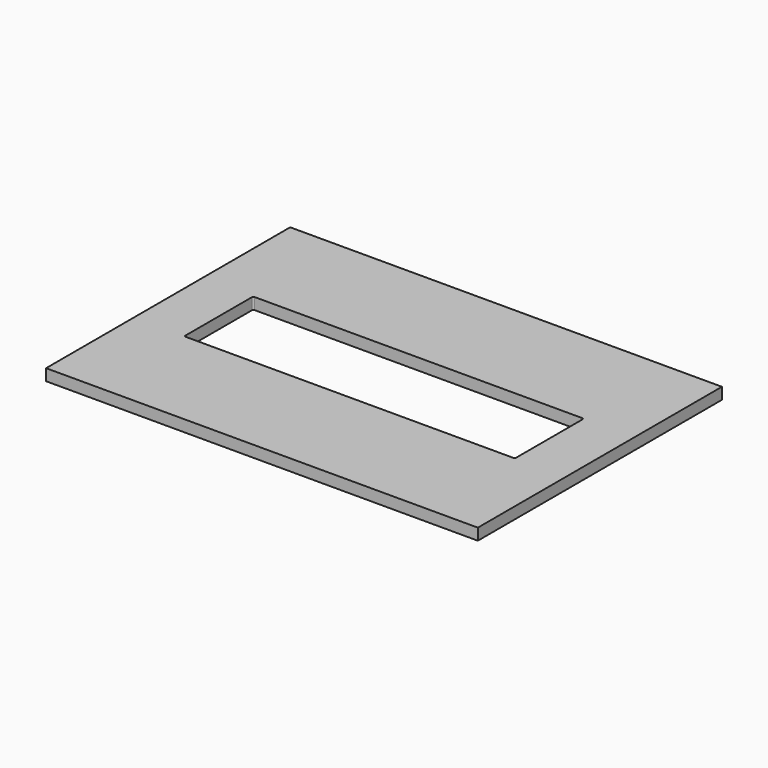
from build123d import *

# Parameters (mm, degrees)
F0_W     = 238.125
F0_H     = 168.275
F1_DEPTH = 6.35
F2_W     = 179.832
F2_H     = 44.958
F3_DEPTH = 25.4
F5_DEPTH = 6.351


# Not quite as in the source:
# - a feature of the source that left no trace in its solid (it failed there, or was rolled back) is left out


with BuildPart() as f1:
    # F0 (on Top) → F1 (new body)
    with BuildSketch(Plane.XY):
        Rectangle(F0_W, F0_H)
    extrude(amount=F1_DEPTH)

    # F2 (on face) → F3 (cut)
    with BuildSketch(Plane.XY.offset(6.35)):
        Rectangle(F2_W, F2_H)
    extrude(amount=-F3_DEPTH, mode=Mode.SUBTRACT)

    # F4 (on face) → F5 (cut, through all)
    with BuildSketch(Plane.XY.offset(6.35)):
        with BuildLine():
            Line((90.3986, 23.749), (-90.3986, 23.749))
            ThreePointArc((-90.3986, 23.749), (-90.9553758795, 23.5183758795), (-91.186, 22.9616))
            Line((-91.186, 22.9616), (-91.186, -22.9616))
            ThreePointArc((-91.186, -22.9616), (-90.9553758795, -23.5183758795), (-90.3986, -23.749))
            Line((-90.3986, -23.749), (90.3986, -23.749))
            ThreePointArc((90.3986, -23.749), (90.9553758795, -23.5183758795), (91.186, -22.9616))
            Line((91.186, -22.9616), (91.186, 22.9616))
            ThreePointArc((91.186, 22.9616), (90.9553758795, 23.5183758795), (90.3986, 23.749))
        make_face()
    extrude(amount=-F5_DEPTH, mode=Mode.SUBTRACT)


solid = f1.part
